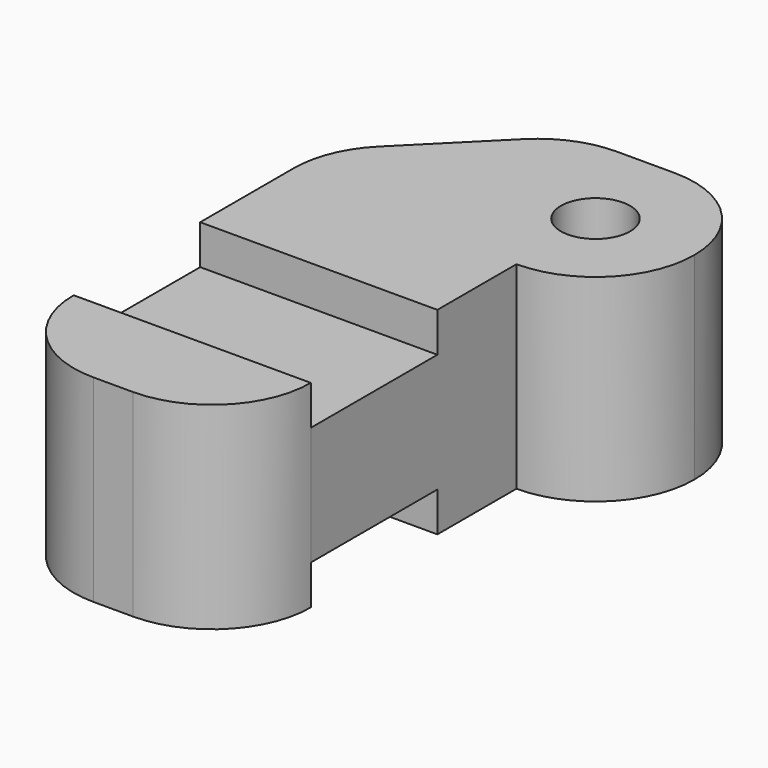
from build123d import *

# Parameters (mm, degrees)
F0_W     = 5
F0_H     = 10
F1_DEPTH = 10
F2_R     = 1.75
F3_DEPTH = 25
F4_W     = 8
F4_H     = 2
F5_DEPTH = 25
F6_R     = 4.99999
F7_SIZE  = 7
F8_R     = 5


# Not quite as in the source:
# - a fillet or chamfer is up to 0.001 mm smaller than in the source, because OpenCascade refuses the exact size


with BuildPart() as f1:
    # F0 (on Top) → F1 (new body)
    with BuildSketch(Plane.XY):
        Polygon((12, 0), (0, 0), (0, -28), (12, -28), (12, -10), align=None)
        with Locations((14.5, -5)):
            Rectangle(F0_W, F0_H)
    extrude(amount=F1_DEPTH)

    # F2 (on face) → F3 (cut)
    with BuildSketch(Plane.XY.offset(10)):
        with Locations((12, -5)):
            Circle(F2_R)
    extrude(amount=-F3_DEPTH, mode=Mode.SUBTRACT)

    # F4 (on face) → F5 (cut)
    with BuildSketch(Plane(origin=(0, 0, 0), x_dir=(0, -1, 0), z_dir=(-1, 0, 0))):
        with Locations((19, 1)):
            Rectangle(F4_W, F4_H)
        with Locations((19, 9)):
            Rectangle(F4_W, F4_H)
    extrude(amount=-F5_DEPTH, mode=Mode.SUBTRACT)

    # F6 (radius 5 in the source; OpenCascade refuses exactly that, so slightly less here)
    f6_edges = [f1.edges().sort_by_distance(p)[0] for p in [
        (12, -28, 5),
        (0, -28, 5),
        (17, 0, 5),
        (17, -10, 5),
    ]]
    fillet(f6_edges, radius=F6_R)

    # F7
    f7_edges = [f1.edges().sort_by_distance(p)[0] for p in [
        (0, 0, 5),
    ]]
    chamfer(f7_edges, length=F7_SIZE)

    # F8
    f8_edges = [f1.edges().sort_by_distance(p)[0] for p in [
        (7, 0, 5),
        (0, -7, 5),
    ]]
    fillet(f8_edges, radius=F8_R)


solid = f1.part
